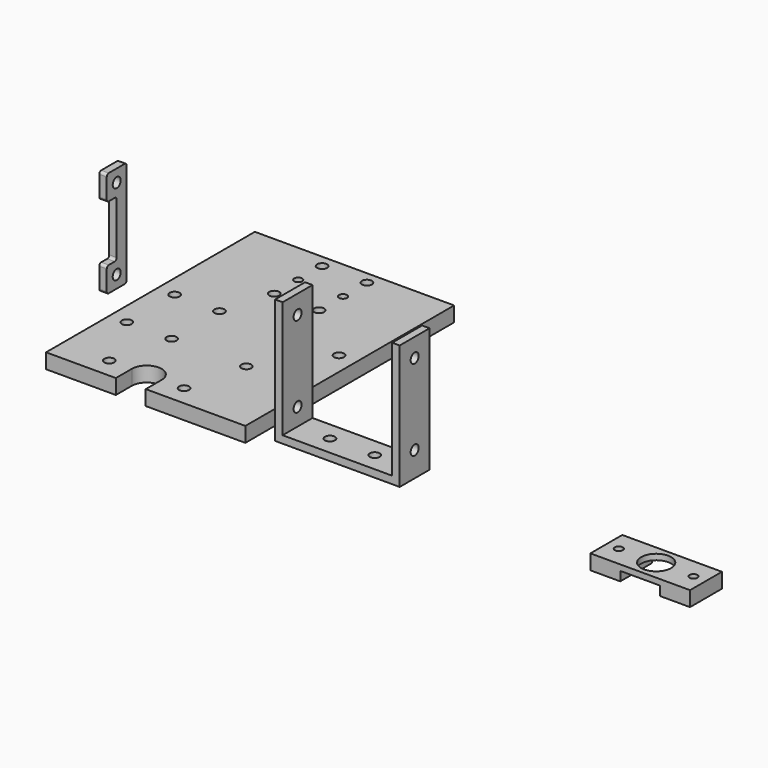
from build123d import *

# Parameters (mm, degrees)
F1_DEPTH  = 15
F3_R      = 2
F4_DEPTH  = 50.001
F2_R      = 2
F5_DEPTH  = 3
F6_R      = 2
F7_DEPTH  = 3
F8_R      = 1
F9_R      = 2
F9_R_2    = 1.6
F10_DEPTH = 6
F11_R     = 2
F12_DEPTH = 6
F14_DEPTH = 16
F15_R     = 1.6
F15_R_2   = 6
F16_DEPTH = 6.001


# Not quite as in the source:
# - a feature names something its author has since deleted; it is built from what else it names


with BuildPart() as f1:
    # F0 (on Front) → F1 (new body)
    with BuildSketch(Plane.XZ):
        Polygon((91.9537246227, 54.5677823946), (91.9537246227, 4.5677823946), (116.9537246227, 4.5677823946), (141.9537246227, 4.5677823946), (141.9537246227, 54.5677823946), (138.9537246227, 54.5677823946), (138.9537246227, 7.5677823946), (116.9537246227, 7.5677823946), (94.9537246227, 7.5677823946), (94.9537246227, 54.5677823946), align=None)
    extrude(amount=-F1_DEPTH)

    # F3 (on face) → F4 (cut, through all)
    with BuildSketch(Plane(origin=(91.9537246227, 0, 0), x_dir=(0, -1, 0), z_dir=(-1, 0, 0))):
        with Locations((-7.5, 47.0677823946)):
            Circle(F3_R)
        with Locations((-7.5, 14.5677823946)):
            Circle(F3_R)
    extrude(amount=-F4_DEPTH, mode=Mode.SUBTRACT)

    # F2 (on face) → F5 (cut, through all)
    with BuildSketch(Plane.XY.offset(7.5677823946)):
        with Locations((107.9537246227, 7.5)):
            Circle(F2_R)
        with Locations((125.9537246227, 7.5)):
            Circle(F2_R)
    extrude(amount=-F5_DEPTH, mode=Mode.SUBTRACT)


with BuildPart() as f7:
    # F6 (on Right) → F7 (new body)
    with BuildSketch(Plane.YZ):
        Polygon((26.6889177019, 26.5677823946), (26.6889177019, 16.5677823946), (36.6889177019, 16.5677823946), (36.6889177019, 59.0677823946), (26.6889177019, 59.0677823946), (26.6889177019, 49.0677823946), (31.6889177019, 49.0677823946), (31.6889177019, 26.5677823946), align=None)
        with Locations((31.6889177019, 21.5677823946)):
            Circle(F6_R, mode=Mode.SUBTRACT)
        with Locations((31.6889177019, 54.0677823946)):
            Circle(F6_R, mode=Mode.SUBTRACT)
    extrude(amount=F7_DEPTH)

    # F8
    f8_edges = [f7.edges().sort_by_distance(p)[0] for p in [
        (1.5, 26.688918, 26.567782),
        (1.5, 26.688918, 16.567782),
        (1.5, 36.688918, 16.567782),
        (1.5, 31.688918, 26.567782),
        (1.5, 31.688918, 49.067782),
        (1.5, 26.688918, 59.067782),
        (1.5, 36.688918, 59.067782),
        (1.5, 26.688918, 49.067782),
    ]]
    fillet(f8_edges, radius=F8_R)


with BuildPart() as f10:
    # F9 (on Top) → F10 (new body)
    with BuildSketch(Plane.XY):
        with BuildLine():
            Line((0, 104.75), (0, 0))
            Line((0, 0), (28, 0))
            Line((28, 0), (28, 8))
            ThreePointArc((28, 8), (34, 14), (40, 8))
            Line((40, 8), (40, 0))
            Line((40, 0), (80, 0))
            Line((80, 0), (80, 104.75))
            Line((80, 104.75), (0, 104.75))
        make_face()
        with Locations((19, 8)):
            Circle(F9_R, mode=Mode.SUBTRACT)
        with Locations((7, 31.75)):
            Circle(F9_R, mode=Mode.SUBTRACT)
        with Locations((25, 31.75)):
            Circle(F9_R, mode=Mode.SUBTRACT)
        with Locations((49, 8)):
            Circle(F9_R, mode=Mode.SUBTRACT)
        with Locations((55, 31.75)):
            Circle(F9_R, mode=Mode.SUBTRACT)
        with Locations((73, 31.75)):
            Circle(F9_R, mode=Mode.SUBTRACT)
        with Locations((7, 55.75)):
            Circle(F9_R, mode=Mode.SUBTRACT)
        with Locations((25, 55.75)):
            Circle(F9_R, mode=Mode.SUBTRACT)
        with Locations((31, 75.75)):
            Circle(F9_R, mode=Mode.SUBTRACT)
        with Locations((31, 87.75)):
            Circle(F9_R_2, mode=Mode.SUBTRACT)
        with Locations((31, 99.75)):
            Circle(F9_R, mode=Mode.SUBTRACT)
        with Locations((55, 55.75)):
            Circle(F9_R, mode=Mode.SUBTRACT)
        with Locations((49, 75.75)):
            Circle(F9_R, mode=Mode.SUBTRACT)
        with Locations((73, 55.75)):
            Circle(F9_R, mode=Mode.SUBTRACT)
        with Locations((49, 87.75)):
            Circle(F9_R_2, mode=Mode.SUBTRACT)
        with Locations((49, 99.75)):
            Circle(F9_R, mode=Mode.SUBTRACT)
    extrude(amount=F10_DEPTH)


with BuildPart() as f12:
    # F11 (on Top) → F12 (new body)
    with BuildSketch(Plane.XY):
        with BuildLine():
            Line((104.3827744635, 71.6418235004), (95.3343725204, 71.6418235004))
            Line((95.3343725204, 71.6418235004), (95.3343725204, 61.6418235004))
            Line((95.3343725204, 61.6418235004), (115.3343725204, 61.6418235004))
            Line((115.3343725204, 61.6418235004), (115.3343725204, 66.8918235004))
            ThreePointArc((115.3343725204, 66.8918235004), (109.3657043273, 68.1304645559), (104.3827744635, 71.6418235004))
        make_face()
        with Locations((100.3343725204, 66.6418235004)):
            Circle(F11_R, mode=Mode.SUBTRACT)
        with BuildLine():
            ThreePointArc((126.2859705774, 71.6418235004), (121.3030407136, 68.1304645559), (115.3343725204, 66.8918235004))
            Line((115.3343725204, 66.8918235004), (115.3343725204, 61.6418235004))
            Line((115.3343725204, 61.6418235004), (135.3343725204, 61.6418235004))
            Line((135.3343725204, 61.6418235004), (135.3343725204, 71.6418235004))
            Line((135.3343725204, 71.6418235004), (126.2859705774, 71.6418235004))
        make_face()
        with Locations((130.3343725204, 66.6418235004)):
            Circle(F11_R, mode=Mode.SUBTRACT)
    extrude(amount=F12_DEPTH)


with BuildPart() as f14:
    # F13 (on Front) → F14 (new body)
    with BuildSketch(Plane.XZ):
        Polygon((218.5050100088, 6), (218.5050100088, 0), (230.5050100088, 0), (230.5050100088, 3.7), (246.5050100088, 3.7), (246.5050100088, 0), (258.5050100088, 0), (258.5050100088, 6), align=None)
    extrude(amount=-F14_DEPTH)

    # F15 (on face) → F16 (cut, through all)
    with BuildSketch(Plane.XY.offset(6)):
        with Locations((223.5050100088, 8)):
            Circle(F15_R)
        with Locations((238.5050100088, 8)):
            Circle(F15_R_2)
        with Locations((253.5050100088, 8)):
            Circle(F15_R)
    extrude(amount=-F16_DEPTH, mode=Mode.SUBTRACT)


solid = Compound([f1.part, f7.part, f10.part, f14.part])
